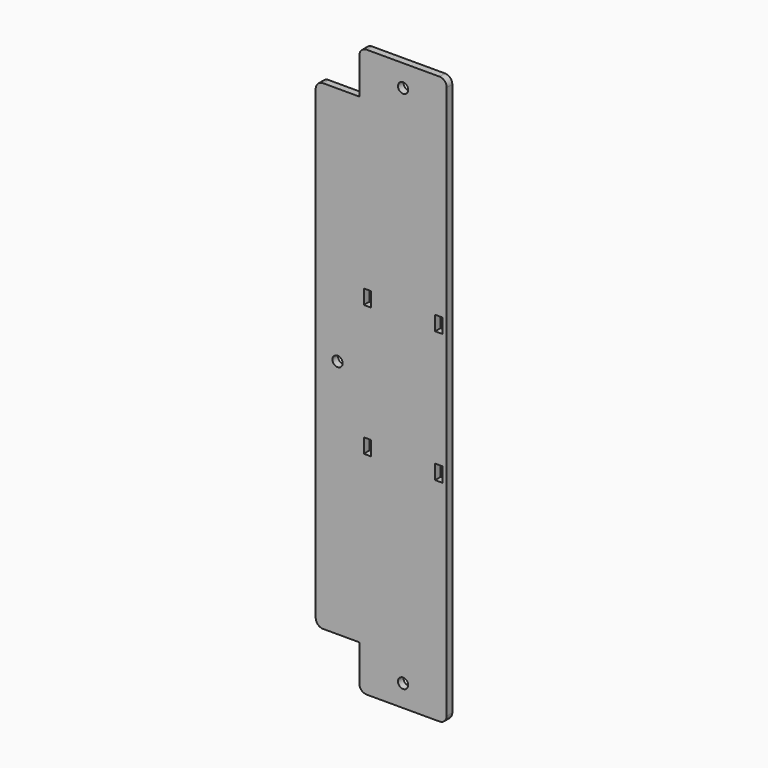
from build123d import *

# Parameters (mm, degrees)
F1_W     = 5
F1_H     = 10
F1_R     = 3.5
F2_DEPTH = 4.7625


# Not quite as in the source:
# - a length typed as a fraction of an inch, garbled in the dataset ("3 / 203.2 mm" for 3/8 in), is restored


with BuildPart() as f2:
    # F1 (on Front) → F2 (new body)
    with BuildSketch(Plane.XZ):
        with BuildLine():
            ThreePointArc((-5, 0), (-1.4644660941, 1.4644660941), (0, 5))
            Line((0, 5), (0, 385))
            ThreePointArc((0, 385), (-1.4644660941, 388.5355339059), (-5, 390))
            Line((-5, 390), (-55, 390))
            ThreePointArc((-55, 390), (-58.5355339059, 388.5355339059), (-60, 385))
            Line((-60, 385), (-60, 360))
            Line((-60, 360), (-85, 360))
            ThreePointArc((-85, 360), (-88.5355339059, 358.5355339059), (-90, 355))
            Line((-90, 355), (-90, 35))
            ThreePointArc((-90, 35), (-88.5355339059, 31.4644660941), (-85, 30))
            Line((-85, 30), (-60, 30))
            Line((-60, 30), (-60, 5))
            ThreePointArc((-60, 5), (-58.5355339059, 1.4644660941), (-55, 0))
            Line((-55, 0), (-5, 0))
        make_face()
        with Locations((-54.5, 150)):
            Rectangle(F1_W, F1_H, mode=Mode.SUBTRACT)
        with Locations((-30, 15)):
            Circle(F1_R, mode=Mode.SUBTRACT)
        with Locations((-5.5, 150)):
            Rectangle(F1_W, F1_H, mode=Mode.SUBTRACT)
        with Locations((-75, 195)):
            Circle(F1_R, mode=Mode.SUBTRACT)
        with Locations((-54.5, 240)):
            Rectangle(F1_W, F1_H, mode=Mode.SUBTRACT)
        with Locations((-5.5, 240)):
            Rectangle(F1_W, F1_H, mode=Mode.SUBTRACT)
        with Locations((-30, 375)):
            Circle(F1_R, mode=Mode.SUBTRACT)
    extrude(amount=F2_DEPTH)


solid = f2.part
